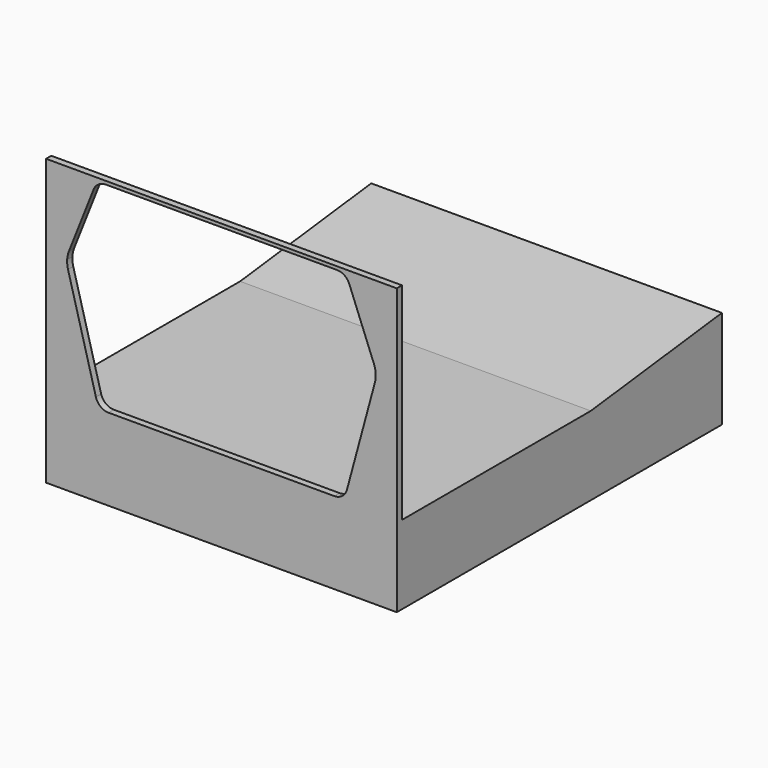
from build123d import *

# Parameters (mm, degrees)
F0_W     = 1358.9
F0_H     = 635
F0_H_2   = 939.8
F1_DEPTH = 304.8
F2_DEPTH = 76.2
F3_SIZE2 = 76.19999
F3_SIZE  = 634.99999
F4_W     = 1358.9
F4_H     = 800.1
F5_DEPTH = 25.4


# Not quite as in the source:
# - a fillet or chamfer is up to 0.001 mm smaller than in the source, because OpenCascade refuses the exact size


with BuildPart() as f1:
    # F0 (on Top) → F1 (new body)
    with BuildSketch(Plane.XY):
        with Locations((679.45, 1257.3)):
            Rectangle(F0_W, F0_H)
        with Locations((679.45, 469.9)):
            Rectangle(F0_W, F0_H_2)
    extrude(amount=-F1_DEPTH)

    # F0 (on Top) → F2 (join)
    with BuildSketch(Plane.XY):
        with Locations((679.45, 1257.3)):
            Rectangle(F0_W, F0_H)
    extrude(amount=F2_DEPTH)

    # F3 (size 635 and 76.2 in the source; OpenCascade refuses exactly that, so slightly less here)
    f3_edges = [f1.edges().sort_by_distance(p)[0] for p in [
        (679.45, 939.8, 76.2),
    ]]
    f3_side = f1.faces().sort_by_distance((679.45, 1257.3, 76.2))[0]
    chamfer(f3_edges, length=F3_SIZE, length2=F3_SIZE2, reference=f3_side)

    # F4 (on face) → F5 (join)
    with BuildSketch(Plane.XZ):
        with Locations((679.45, 400.05)):
            Rectangle(F4_W, F4_H)
        with BuildLine():
            Line((1116.8070589646, 12.7), (242.0929410354, 12.7))
            ThreePointArc((242.0929410354, 12.7), (211.2114924509, 23.1642077886), (193.0524806695, 50.2458215227))
            Line((193.0524806695, 50.2458215227), (84.9974320158, 450.0495015416))
            ThreePointArc((84.9974320158, 450.0495015416), (82.0087933028, 466.189437514), (81.6581746464, 482.6))
            ThreePointArc((81.6581746464, 482.6), (83.887579714, 498.5521883341), (88.6100008594, 513.9515811185))
            Line((88.6100008594, 513.9515811185), (184.1425076023, 755.2968613112))
            ThreePointArc((184.1425076023, 755.2968613112), (202.8211285229, 778.6145245993), (231.3766835464, 787.4))
            Line((231.3766835464, 787.4), (1127.5233164536, 787.4))
            ThreePointArc((1127.5233164536, 787.4), (1156.0788714771, 778.6145245993), (1174.7574923977, 755.2968613112))
            Line((1174.7574923977, 755.2968613112), (1270.2899991406, 513.9515811185))
            ThreePointArc((1270.2899991406, 513.9515811185), (1275.012420286, 498.5521883341), (1277.2418253536, 482.6))
            ThreePointArc((1277.2418253536, 482.6), (1276.8912066972, 466.189437514), (1273.9025679842, 450.0495015416))
            Line((1273.9025679842, 450.0495015416), (1165.8475193305, 50.2458215227))
            ThreePointArc((1165.8475193305, 50.2458215227), (1147.6885075491, 23.1642077886), (1116.8070589646, 12.7))
        make_face(mode=Mode.SUBTRACT)
    extrude(amount=-F5_DEPTH)


solid = f1.part
